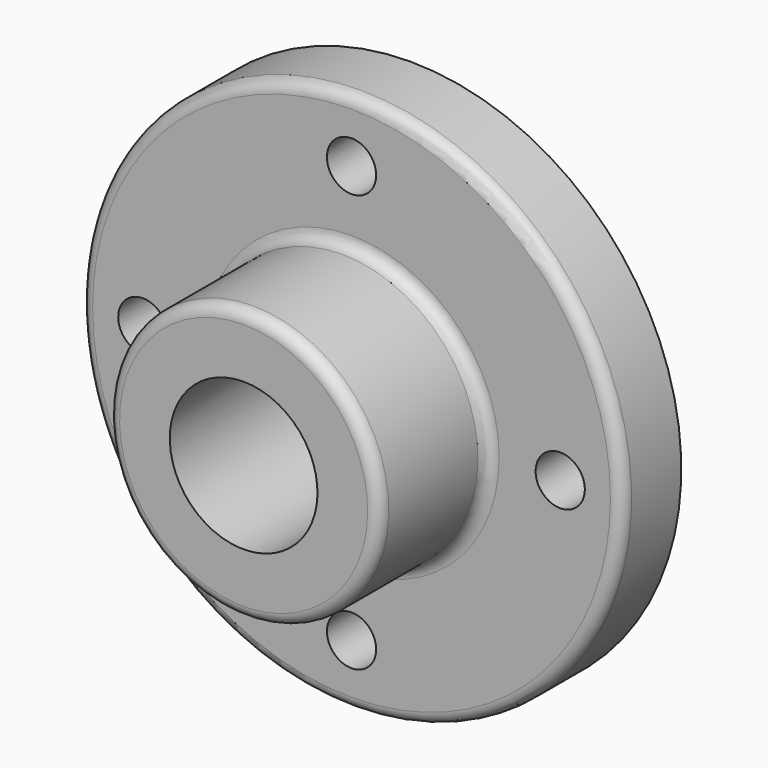
from build123d import *

# Parameters (mm, degrees)
F2_R            = 6.35
F3_DEPTH        = 19.051
F3_COPIES_COUNT = 4
F4_R            = 3.048


# Not quite as in the source:
# - a pattern or mirror of a feature is missing from the dataset's text; its kind, count and spacing are read off the source's solid


with BuildPart() as f1:
    # F0 (on Right) → F1 (revolve)
    with BuildSketch(Plane.YZ):
        Polygon((-53.848, 19.05), (0, 19.05), (0, 69.85), (-19.05, 69.85), (-19.05, 35.052), (-53.848, 35.052), align=None)
    revolve(axis=Axis((0, -0.6338636002, 0), (0, 1, 0)))

    # F2 (on face) → F3 (cut, through all)
    with BuildSketch(Plane.XZ.offset(19.05)):
        with Locations((0, 53.848)):
            Circle(F2_R)
    f3 = extrude(amount=-F3_DEPTH, mode=Mode.SUBTRACT)

    # F3_copies: F3 ×4 about axis
    f3_copies_axis = Axis((0, 0, 0), (0, 1, 0))
    for i in range(1, F3_COPIES_COUNT):
        add(f3.rotate(f3_copies_axis, i * 360 / F3_COPIES_COUNT), mode=Mode.SUBTRACT)

    # F4
    f4_edges = [f1.edges().sort_by_distance(p)[0] for p in [
        (0, -19.05, -69.85),
        (0, -53.848, -35.052),
        (0, -19.05, -35.052),
    ]]
    fillet(f4_edges, radius=F4_R)


solid = f1.part
